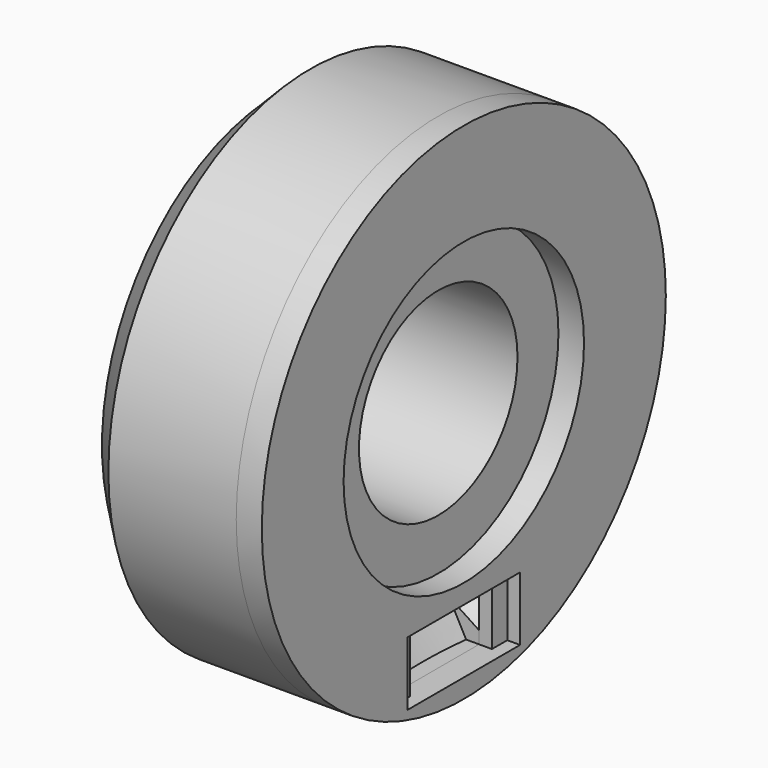
from build123d import *

# Parameters (mm, degrees)
F0_W        = 25
F0_H        = 2
F2_SIZE     = 5
F3_R        = 39.5
F3_R_2      = 23.5068353711
F4_DEPTH    = 4
F5_W        = 8
F5_H        = 10
F6_DEPTH    = 4.5
F5_W_2      = 3
F7_DEPTH    = 2
F8_T4_ANGLE = 68.4635032376


# Not quite as in the source:
# - a fillet or chamfer that OpenCascade refuses, or shapes differently, is made with other operations: its cross-section is extruded or revolved along the edge and cut away or added


with BuildPart() as f1:
    # F0 (on Top) → F1 (revolve)
    with BuildSketch(Plane.XY):
        with Locations((0, 16.5)):
            Rectangle(F0_W, F0_H)
        Polygon((12.5, 25.5), (-12.5, 17.5), (12.5, 17.5), align=None)
    revolve(axis=Axis((0, 0, 0), (-1, 0, 0)))


with BuildPart() as f1b:
    # F0 (on Top) → F1, piece 2 (revolve)
    with BuildSketch(Plane.XY):
        Polygon((-12.5, 22.5), (-12.5, 19.5), (12.5, 35.4886714636), (12.5, 39.5), (-12.5, 39.5), (-12.5, 27.5), (-8.5, 27.5), (-8.5, 22.5), align=None)
    revolve(axis=Axis((0, 0, 0), (-1, 0, 0)))

    # F2
    f2_edges = [f1b.edges().sort_by_distance(p)[0] for p in [
        (-12.5, -39.5, 0),
    ]]
    chamfer(f2_edges, length=F2_SIZE)


with BuildPart() as f4:
    # F3 (on face) → F4 (new body)
    with BuildSketch(Plane.YZ.offset(12.5)):
        Circle(F3_R)
        Circle(F3_R_2, mode=Mode.SUBTRACT)
    extrude(amount=F4_DEPTH)


with BuildPart() as f6_tool:
    # F5 (on face) → F6 (new body)
    with BuildSketch(Plane.YZ.offset(16.5)):
        with Locations((-4, -31.5034176856)):
            Rectangle(F5_W, F5_H)
        with Locations((4, -31.5034176856)):
            Rectangle(F5_W, F5_H)
    extrude(amount=-F6_DEPTH)


with BuildPart() as f1b_1:
    add(f1b.part)

    # F6: cut by f6_tool
    add(f6_tool.part, mode=Mode.SUBTRACT)

    # F8: chamfer of 5 on 1 edges, made by hand


with BuildPart() as f4_1:
    add(f4.part)

    # F6: cut by f6_tool
    add(f6_tool.part, mode=Mode.SUBTRACT)

    # F5 (on face) → F7 (cut)
    with BuildSketch(Plane.YZ.offset(16.5)):
        with Locations((-9.5, -31.5034176856)):
            Rectangle(F5_W_2, F5_H)
        with Locations((9.5, -31.5034176856)):
            Rectangle(F5_W_2, F5_H)
    extrude(amount=-F7_DEPTH, mode=Mode.SUBTRACT)


with BuildPart() as f8_tool2:
    # F8_s3 → F8_t4 (revolve)
    with BuildSketch(Plane(origin=(0, 0, 0), x_dir=(1, 0, 0), z_dir=(0, -0.8267689574, 0.562541635))):
        Polygon((7.7877765933, -32.474983787), (12, -40.1688980343), (12, -35.1688980343), align=None)
    revolve(axis=Axis((12, 0, 0), (1, 0, 0)), revolution_arc=F8_T4_ANGLE)

    split(bisect_by=Plane.XZ.offset(8), keep=Keep.BOTTOM)

    split(bisect_by=Plane.XY.offset(-36.5034176856), keep=Keep.TOP)

    split(bisect_by=Plane.XZ.offset(-8), keep=Keep.TOP)


with BuildPart() as f1b_2:
    add(f1b_1.part)

    # F8_t1: cut F8_tool2
    add(f8_tool2.part, mode=Mode.SUBTRACT)


solid = Compound([f1.part, f4_1.part, f1b_2.part])
